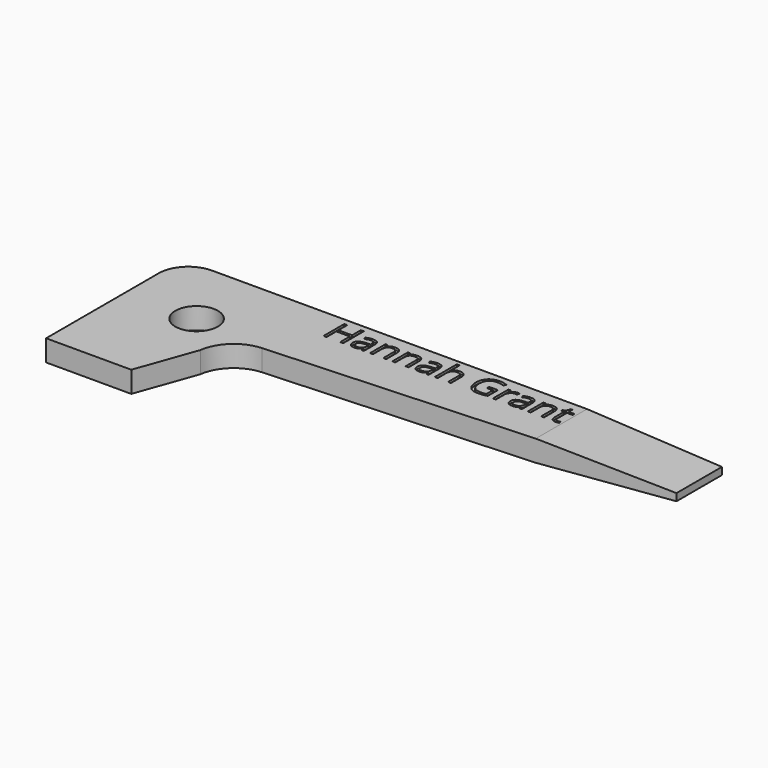
from build123d import *

# Parameters (mm, degrees)
F1_DEPTH     = 2.38125
F2_R         = 2.3876
F3_DEPTH     = 25.4
F5_DEPTH     = 25.4
F6_TEXT_SIZE = 4.0567573344
F7_DEPTH     = 0.254


# Not quite as in the source:
# - Text() gives the source's letters only with a copy of the font that has no kerning and outlines rounded to 1/6400 em; it was checked with that copy


with BuildPart() as f1:
    # F0 (on Top) → F1 (new body)
    with BuildSketch(Plane.XY):
        with BuildLine():
            Line((60.325, 19.05), (3.302, 19.05))
            ThreePointArc((3.302, 19.05), (0.9671334085, 18.0828665915), (0, 15.748))
            Line((0, 15.748), (0, 0))
            Line((0, 0), (9.525, 0))
            Line((9.525, 0), (11.9123317803, 6.6641346697))
            ThreePointArc((11.9123317803, 6.6641346697), (13.2332907685, 9.2094144639), (15.875, 10.3251))
            Line((15.875, 10.3251), (60.325, 12.7))
            Line((60.325, 12.7), (60.325, 19.05))
        make_face()
    extrude(amount=F1_DEPTH)

    # F2 (on face) → F3 (cut)
    with BuildSketch(Plane.XY.offset(2.38125)):
        with Locations((7.9502, 11.0998)):
            Circle(F2_R)
    extrude(amount=-F3_DEPTH, mode=Mode.SUBTRACT)

    # F4 (on face) → F5 (cut)
    with BuildSketch(Plane(origin=(0, 19.05, 0), x_dir=(-1, 0, 0), z_dir=(0, 1, 0))):
        Polygon((-60.325, 1.59385), (-45.2374, 2.38125), (-60.325, 2.38125), align=None)
        Polygon((-45.2374, 0), (-60.325, 0.7874), (-60.325, 0), align=None)
    extrude(amount=-F5_DEPTH, mode=Mode.SUBTRACT)

    # F6 (on face) → F7 (cut)
    with BuildSketch(Plane.XY.offset(2.38125)):
        with Locations((18.2434831499, 15.4719455429)):
            Text('Hannah Grant', F6_TEXT_SIZE, font='Open Sans', text_align=(TextAlign.LEFT, TextAlign.BOTTOM))
    extrude(amount=-F7_DEPTH, mode=Mode.SUBTRACT)


solid = f1.part
